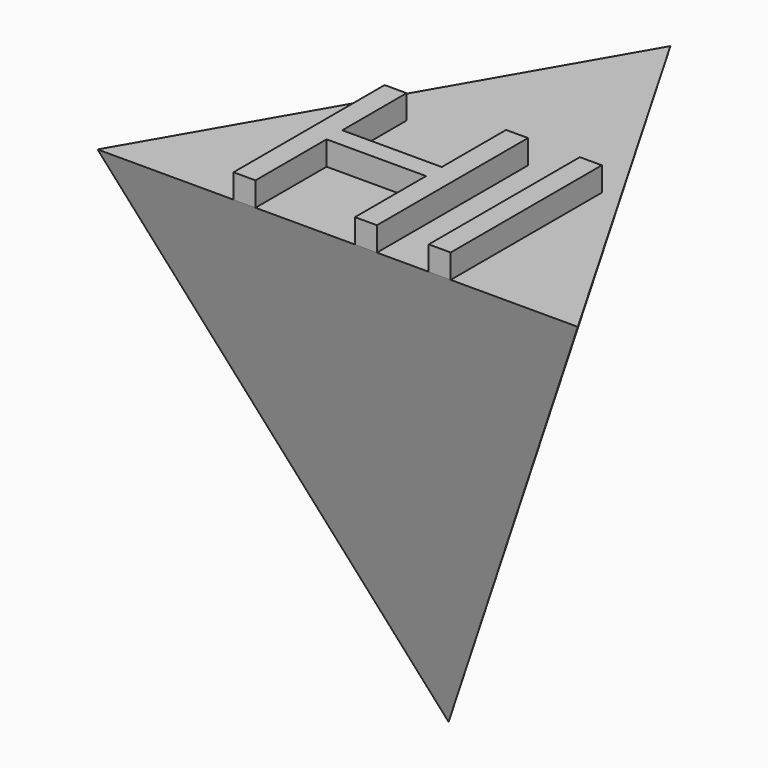
from build123d import *

# Parameters (mm, degrees)
F4_TEXT_SIZE = 27.8710898168
F5_DEPTH     = 2.54


# Not quite as in the source:
# - Text() gives the source's letters only with a copy of the font that has no kerning and outlines rounded to 1/6400 em; it was checked with that copy


with BuildPart() as f3:
    # F2 (on offset) → F3 section 0
    with BuildSketch(Plane.XY.offset(50.8), mode=Mode.PRIVATE) as f3_s0:
        Polygon((-25.2948867737, -14.6040096879), (25.2948867737, -14.6040096879), (0, 29.2080193758), align=None)
    loft([f3_s0.sketch, Vertex(0, 0, 0)])

    # F4 (on face) → F5 (join)
    with BuildSketch(Plane.XY.offset(50.8)):
        with Locations((-13.7090923037, -14.6040096879)):
            Text('HI', F4_TEXT_SIZE, font='Open Sans', text_align=(TextAlign.LEFT, TextAlign.BOTTOM))
    extrude(amount=F5_DEPTH)


solid = f3.part
